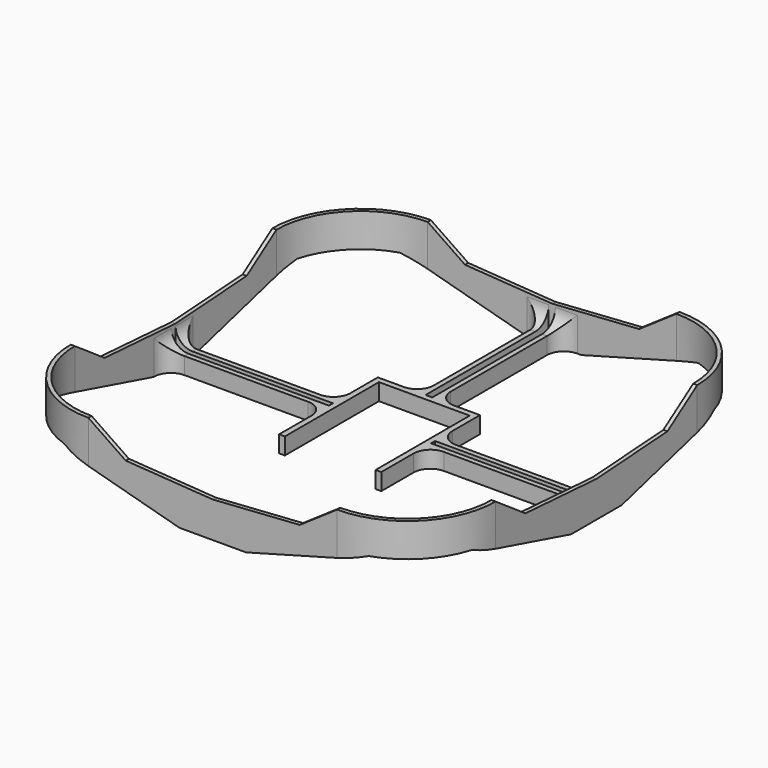
from build123d import *

# Parameters (mm, degrees)
F1_DEPTH  = 20
F0_W      = 1.5
F0_H      = 45.8000004292
F0_W_2    = 46.8000004292
F0_H_2    = 1.5
F2_DEPTH  = 5
F3_R      = 5
F5_DEPTH  = 150.7
F7_DEPTH  = 137.6
F13_DEPTH = 60
F14_DEPTH = 56.1
F20_DEPTH = 72.8
F21_DEPTH = 71.7


with BuildPart() as f1:
    # F0 (on Top) → F1 (new body)
    with BuildSketch(Plane.XY):
        with BuildLine():
            Line((37, 63.7), (-37, 63.7))
            ThreePointArc((-37, 63.7), (-55.5261976671, 56.0261976671), (-63.2, 37.5))
            Line((-63.2, 37.5), (-63.2, -37.5))
            ThreePointArc((-63.2, -37.5), (-55.5261976671, -56.0261976671), (-37, -63.7))
            Line((-37, -63.7), (37, -63.7))
            ThreePointArc((37, -63.7), (55.5261976671, -56.0261976671), (63.2, -37.5))
            Line((63.2, -37.5), (63.2, 37.5))
            ThreePointArc((63.2, 37.5), (55.5261976671, 56.0261976671), (37, 63.7))
        make_face()
        with BuildLine():
            ThreePointArc((-62, 37.5), (-54.6776695297, 55.1776695297), (-37, 62.5))
            Line((-37, 62.5), (-2.5, 62.5))
            Line((-2.5, 62.5), (-1, 62.5))
            Line((-1, 62.5), (1, 62.5))
            Line((1, 62.5), (2.5, 62.5))
            Line((2.5, 62.5), (37, 62.5))
            ThreePointArc((37, 62.5), (54.6776695297, 55.1776695297), (62, 37.5))
            Line((62, 37.5), (62, 1.5))
            Line((62, 1.5), (62, 0))
            Line((62, 0), (62, -1.5))
            Line((62, -1.5), (62, -3))
            Line((62, -3), (62, -37.5))
            ThreePointArc((62, -37.5), (54.6776695297, -55.1776695297), (37, -62.5))
            Line((37, -62.5), (-37, -62.5))
            ThreePointArc((-37, -62.5), (-54.6776695297, -55.1776695297), (-62, -37.5))
            Line((-62, -37.5), (-62, -3))
            Line((-62, -3), (-62, -1.5))
            Line((-62, -1.5), (-62, 0))
            Line((-62, 0), (-62, 1.5))
            Line((-62, 1.5), (-62, 37.5))
        make_face(mode=Mode.SUBTRACT)
    extrude(amount=F1_DEPTH)

    # F0 (on Top) → F2 (join)
    with BuildSketch(Plane.XY):
        with Locations((1.75, 39.5999997854)):
            Rectangle(F0_W, F0_H)
        Polygon((-1, 16.6999995708), (-2.5, 16.6999995708), (-15.1999995708, 16.6999995708), (-15.1999995708, 1.5), (-15.1999995708, 0), (-15.1999995708, -1.5), (-15.1999995708, -3), (-15.1999995708, -16.6999995708), (-15.1999995708, -20), (-13.5, -20), (-13.5, -15), (-13.5, 15), (13.5, 15), (13.5, -15), (13.5, -20), (15.1999995708, -20), (15.1999995708, -15), (15.1999995708, -3), (15.1999995708, -1.5), (15.1999995708, 0), (15.1999995708, 1.5), (15.1999995708, 16.6999995708), (2.5, 16.6999995708), (1, 16.6999995708), align=None)
        with Locations((-1.75, 39.5999997854)):
            Rectangle(F0_W, F0_H)
        with Locations((-38.5999997854, 0.75)):
            Rectangle(F0_W_2, F0_H_2)
        with Locations((-38.5999997854, -2.25)):
            Rectangle(F0_W_2, F0_H_2)
        with Locations((38.5999997854, 0.75)):
            Rectangle(F0_W_2, F0_H_2)
        with Locations((38.5999997854, -2.25)):
            Rectangle(F0_W_2, F0_H_2)
    extrude(amount=F2_DEPTH)

    # F3
    f3_edges = [f1.edges().sort_by_distance(p)[0] for p in [
        (-2.5, 62.5, 2.5),
        (2.5, 62.5, 2.5),
        (-2.5, 16.7, 2.5),
        (2.5, 16.7, 2.5),
        (62, 1.5, 2.5),
        (15.2, 1.5, 2.5),
        (62, -3, 2.5),
        (15.2, -3, 2.5),
        (-15.2, -3, 2.5),
        (-62, -3, 2.5),
        (-62, 1.5, 2.5),
        (-15.2, 1.5, 2.5),
        (1.75, 62.5, 5),
        (-1.75, 62.5, 5),
        (62, 0.75, 5),
        (62, -2.25, 5),
        (-62, 0.75, 5),
        (-62, -2.25, 5),
    ]]
    fillet(f3_edges, radius=F3_R)

    # F4 (on face) → F5 (cut)
    with BuildSketch(Plane(origin=(0, 63.7, 0), x_dir=(-1, 0, 0), z_dir=(0, 1, 0))):
        Polygon((37, 20), (-37, 20), (-25.8996840566, 12.3994192109), (0, 10.6452321634), (25.8996840566, 12.3994192109), align=None)
    extrude(amount=-F5_DEPTH, mode=Mode.SUBTRACT)

    # F6 (on face) → F7 (cut)
    with BuildSketch(Plane(origin=(-63.2, 0, 0), x_dir=(0, -1, 0), z_dir=(-1, 0, 0))):
        Polygon((37.5, 20), (-37.5, 20), (-26.3996840566, 12.3994192109), (0, 10.6842042878), (26.3996840566, 12.3994192109), align=None)
    extrude(amount=-F7_DEPTH, mode=Mode.SUBTRACT)

    # F12 (on face) → F13 (cut)
    with BuildSketch(Plane(origin=(-74.2462120246, -74.2462120246, 0), x_dir=(-0.7071067812, 0.7071067812, 0), z_dir=(0.7071067812, 0.7071067812, 0))):
        Polygon((-12, 10), (-38.037519902, 0), (38.037519902, 0), (12, 10), (0, 10), align=None)
    extrude(amount=F13_DEPTH, mode=Mode.SUBTRACT)

    # F10 (on face) → F14 (cut)
    with BuildSketch(Plane(origin=(71.6299169342, 71.6299169342, 0), x_dir=(-0.7071067812, 0.7071067812, 0), z_dir=(0.7071067812, 0.7071067812, 0))):
        Polygon((-38.037519902, 0), (0, 0), (0, 10), (-12, 10), align=None)
        Polygon((0, 10), (0, 0), (38.037519902, 0), (12, 10), align=None)
    extrude(amount=-F14_DEPTH, mode=Mode.SUBTRACT)

    # F19 (on face) → F20 (cut)
    with BuildSketch(Plane(origin=(84.1457069612, -84.1457069612, 0), x_dir=(-0.7071067812, -0.7071067812, 0), z_dir=(-0.7071067812, 0.7071067812, 0))):
        Polygon((-12.000480098, 10), (-38.038, 0), (38.037039804, 0), (11.999519902, 10), (-0.000480098, 10), align=None)
    extrude(amount=F20_DEPTH, mode=Mode.SUBTRACT)

    # F18 (on face) → F21 (cut)
    with BuildSketch(Plane(origin=(-82.0243866176, 82.0243866176, 0), x_dir=(-0.7071067812, -0.7071067812, 0), z_dir=(-0.7071067812, 0.7071067812, 0))):
        Polygon((-12.000480098, 10), (-38.038, 0), (38.037039804, 0), (11.999519902, 10), (-0.000480098, 10), align=None)
    extrude(amount=-F21_DEPTH, mode=Mode.SUBTRACT)


solid = f1.part
